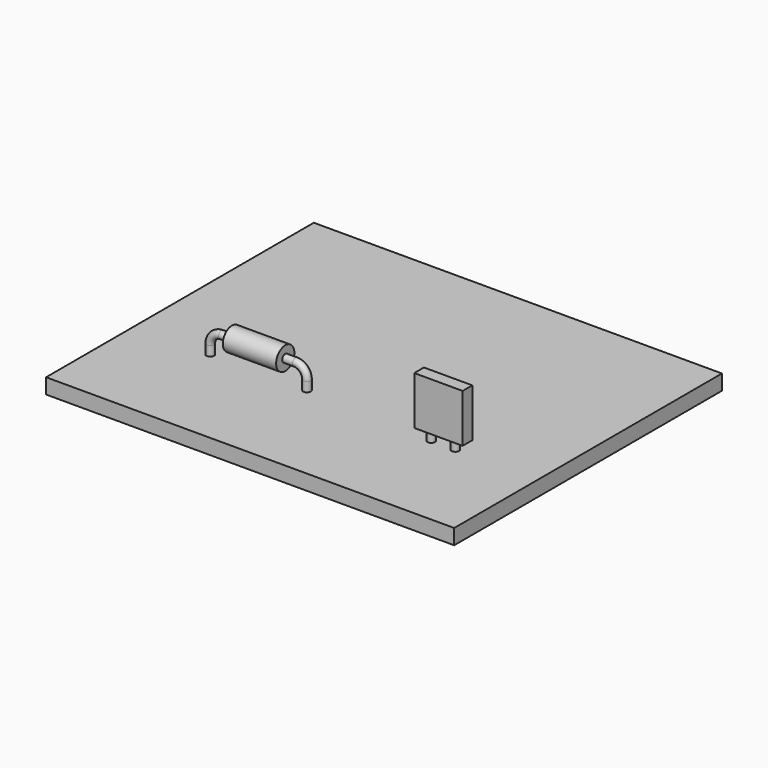
from build123d import *

# Parameters (mm, degrees)
F0_W      = 53.608039394
F0_H      = 43.9585913264
F1_DEPTH  = 2
F2_W      = 7
F2_H      = 1.5
F4_R      = 0.5
F7_R      = 0.15
F10_W     = 6.35
F10_H     = 6.35
F11_DEPTH = 1.5875
F12_R     = 0.5


# Not quite as in the source:
# - a length typed as a fraction of an inch, garbled in the dataset ("3 / 203.2 mm" for 3/8 in), is restored


with BuildPart() as f1:
    # F0 (on Top) → F1 (new body)
    with BuildSketch(Plane.XY):
        with Locations((-3.6185430363, 7.5051253516)):
            Rectangle(F0_W, F0_H)
    extrude(amount=F1_DEPTH)


with BuildPart() as f3:
    # F2 (on Front) → F3 (revolve)
    with BuildSketch(Plane.XZ):
        with Locations((-14.0843965262, 5.52)):
            Rectangle(F2_W, F2_H)
    revolve(axis=Axis((-14.0843965262, 0, 4.77), (1, 0, 0)))


with BuildPart() as f6:
    # F6: sweep along a path in F5
    with BuildLine(Plane.XZ) as f6_path:
        Line((-17.5843965262, 4.77), (-18.9343965262, 4.77))
        ThreePointArc((-18.9343965262, 4.77), (-19.995056698, 4.3306601718), (-20.4343965262, 3.27))
        Line((-20.4343965262, 3.27), (-20.4343965262, -1.27))
    # F4 (on face) → F6 (sweep)
    with BuildSketch(Plane(origin=(-17.5843965262, 0, 0), x_dir=(0, -1, 0), z_dir=(-1, 0, 0))):
        with Locations((0, 4.77)):
            Circle(F4_R)
    sweep(path=f6_path.line)

    # F7
    f7_edges = [f6.edges().sort_by_distance(p)[0] for p in [
        (-20.434397, 0.5, -1.27),
    ]]
    fillet(f7_edges, radius=F7_R)


with BuildPart() as f9_1:
    # F9: instance of F6
    add(f6.part.mirror(Plane(origin=(-14.0843965262, 0, 0), x_dir=(0, -1, 0), z_dir=(-1, 0, 0))))


with BuildPart() as f11:
    # F10 (on Front) → F11 (new body)
    with BuildSketch(Plane.XZ):
        with Locations((10.8077574987, 6.445)):
            Rectangle(F10_W, F10_H)
    extrude(amount=F11_DEPTH)


with BuildPart() as f14:
    # F14: sweep along a path in F13
    with BuildLine(Plane.XZ) as f14_path:
        Line((9.2202574987, 3.27), (9.2202574987, -1.27))
    # F12 (on face) → F14 (sweep)
    with BuildSketch(Plane(origin=(0, 0, 3.27), x_dir=(1, 0, 0), z_dir=(0, 0, -1))):
        with Locations((9.2202574987, 0.79375)):
            Circle(F12_R)
        with Locations((12.3952574987, 0.79375)):
            Circle(F12_R)
    sweep(path=f14_path.line)


solid = Compound([f1.part, f3.part, f6.part, f9_1.part, f11.part, f14.part])
